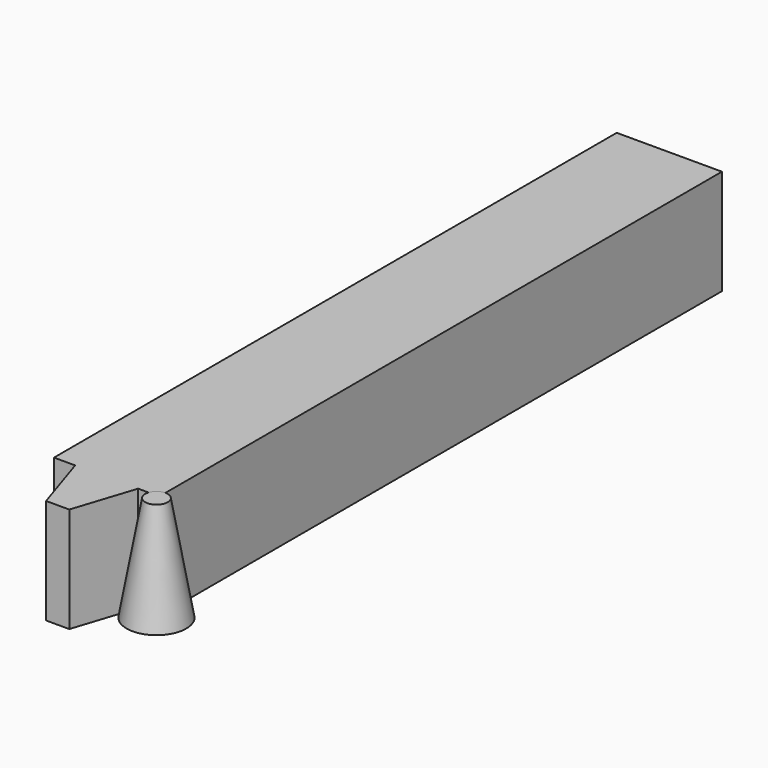
from build123d import *

# Parameters (mm, degrees)
F4_W      = 14.859
F4_H      = 14.859
F5_DEPTH  = 107.95
F10_DEPTH = 14.859


# Not quite as in the source:
# - a length typed as a fraction of an inch, garbled in the dataset ("3 / 203.2 mm" for 3/8 in), is restored


with BuildPart() as f5:
    # F4 (on Front) → F5 (new body)
    with BuildSketch(Plane.XZ):
        with Locations((38.387173794, 26.6289538287)):
            Rectangle(F4_W, F4_H)
    extrude(amount=-F5_DEPTH)

    # F6 (on face) → F10 (cut, through all)
    with BuildSketch(Plane.XY.offset(34.0584538287)):
        Polygon((30.957673794, 0), (36.7481802907, 0), (33.942173794, 8.636), (30.957673794, 8.636), align=None)
        Polygon((42.832173794, 8.636), (40.0261672974, 0), (45.816673794, 0), (45.816673794, 8.636), align=None)
    extrude(amount=-F10_DEPTH, mode=Mode.SUBTRACT)


with BuildPart() as f9:
    # F8 (on face) → F9 (revolve)
    with BuildSketch(Plane.YZ.offset(45.816673794)):
        Polygon((12.3529781278, 19.1994538287), (9.7329355214, 34.0584538287), (8.1454355214, 34.0584538287), (8.1454355214, 19.1994538287), align=None)
    revolve(axis=Axis((45.816673794, 8.1454355214, 26.6289538287), (0, 0, -1)))


solid = Compound([f5.part, f9.part])
